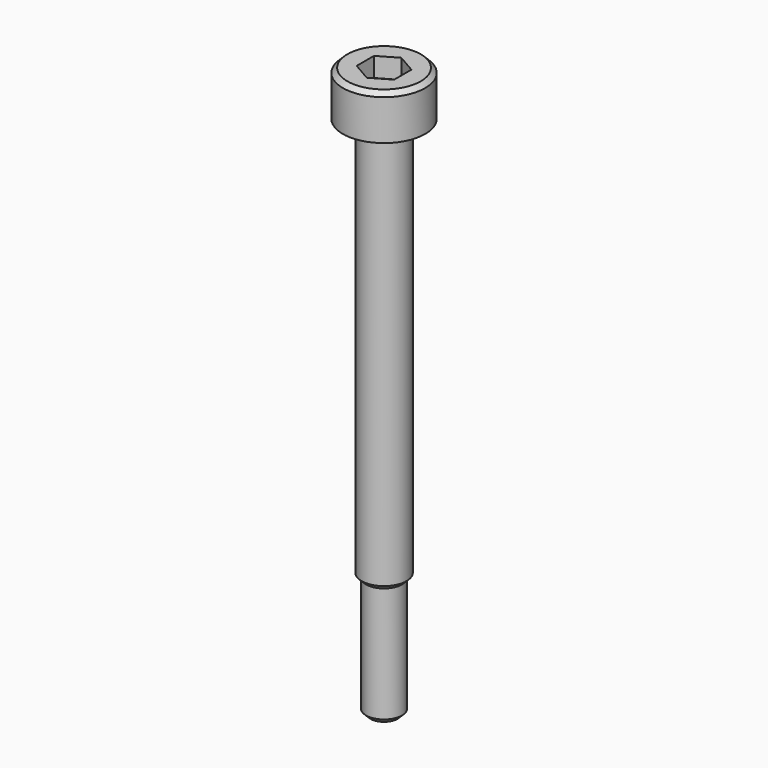
from build123d import *

# Parameters (mm, degrees)
F3_R       = 1.5
F4_DEPTH   = 27
F5_R       = 1.2
F6_DEPTH   = 8
F3_R_2     = 2.75
F4_FACE1_R = 1.5
F7_DEPTH   = 3
F8_SIZE    = 0.29999
F10_DEPTH  = 1.3


# Not quite as in the source:
# - a fillet or chamfer is up to 0.001 mm smaller than in the source, because OpenCascade refuses the exact size


with BuildPart() as f4:
    # F3 (on Top) → F4 (new body)
    with BuildSketch(Plane.XY):
        Circle(F3_R)
    extrude(amount=-F4_DEPTH)

    # F5 (on face) → F6 (join)
    with BuildSketch(Plane(origin=(0, 0, -27), x_dir=(1, 0, 0), z_dir=(0, 0, -1))):
        Circle(F5_R)
    extrude(amount=F6_DEPTH)

    # F3 (on Top) + F4_face1 (on face) → F7 (join)
    with BuildSketch(Plane.XY):
        Circle(F3_R_2)
        Circle(F3_R, mode=Mode.SUBTRACT)
    with BuildSketch(Plane.XY):
        Circle(F4_FACE1_R)
    extrude(amount=F7_DEPTH)

    # F8 (size 0.3 in the source; OpenCascade refuses exactly that, so slightly less here)
    f8_edges = [f4.edges().sort_by_distance(p)[0] for p in [
        (-1.5, 0, -27),
        (-2.75, 0, 3),
        (-1.2, 0, -35),
    ]]
    chamfer(f8_edges, length=F8_SIZE)

    # F9 (on face) → F10 (cut)
    with BuildSketch(Plane.XY.offset(3)):
        Polygon((1.25, -0.7216878365), (1.25, 0.7216878365), (0, 1.443375673), (-1.25, 0.7216878365), (-1.25, -0.7216878365), (0, -1.443375673), align=None)
    extrude(amount=-F10_DEPTH, mode=Mode.SUBTRACT)


solid = f4.part
